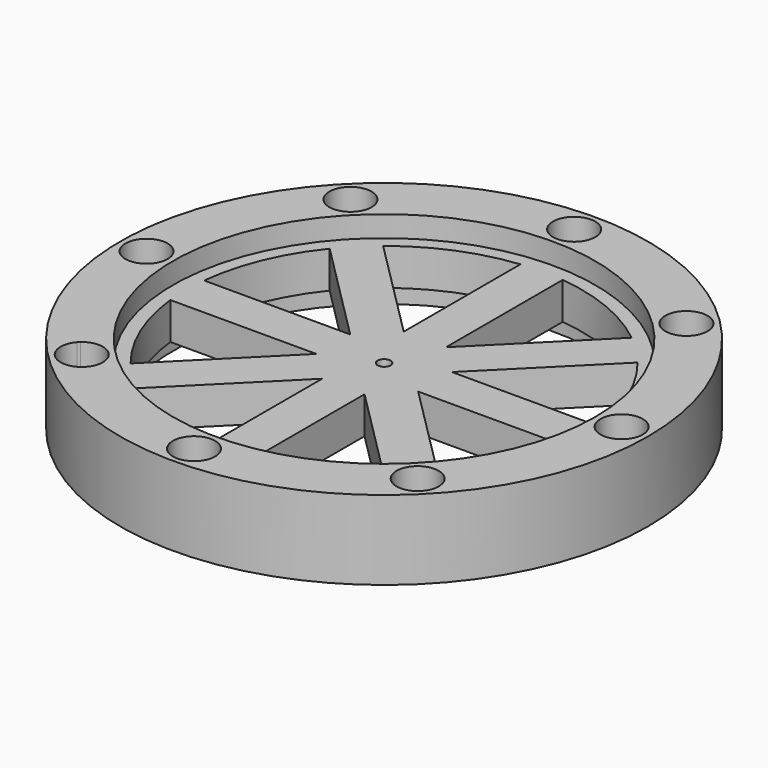
from build123d import *

# Parameters (mm, degrees)
F0_R     = 63.5
F0_R_2   = 5.08
F0_R_3   = 1.5621
F1_DEPTH = 19.05
F2_R     = 50.8
F2_R_2   = 1.5621
F3_DEPTH = 5.08
F4_R     = 50.8
F4_R_2   = 1.5621
F5_DEPTH = 5.08


with BuildPart() as f1:
    # F0 (on Top) → F1 (new body)
    with BuildSketch(Plane.XY):
        Circle(F0_R)
        with BuildLine():
            ThreePointArc((-43.7932900831, -36.6206979979), (-36.8187913893, -44.0029962675), (-44.2020942404, -37.0295610466))
            Line((-44.2020942404, -37.0295610466), (-43.7932900831, -36.6206979979))
        make_face(mode=Mode.SUBTRACT)
        with BuildLine():
            Line((-5.08, -12.2641944787), (-5.08, -47.3532915963))
            Line((-5.08, -47.3532915963), (-5.08, -50.545361805))
            ThreePointArc((-5.08, -50.545361805), (-19.4403188674, -46.9330800431), (-32.1488664849, -39.3330698488))
            Line((-32.1488664849, -39.3330698488), (-29.8917324097, -37.0759350327))
            Line((-29.8917324097, -37.0759350327), (-5.08, -12.2641944787))
        make_face(mode=Mode.SUBTRACT)
        with BuildLine():
            ThreePointArc((-39.328136569, -32.154901244), (-46.9315884756, -19.4439194393), (-50.545361805, -5.08))
            Line((-50.545361805, -5.08), (-47.3532915963, -5.08))
            Line((-47.3532915963, -5.08), (-12.2571351119, -5.08))
            Line((-12.2571351119, -5.08), (-37.0711843605, -29.8976239041))
            Line((-37.0711843605, -29.8976239041), (-39.328136569, -32.154901244))
        make_face(mode=Mode.SUBTRACT)
        with Locations((0, -57.15)):
            Circle(F0_R_2, mode=Mode.SUBTRACT)
        with BuildLine():
            ThreePointArc((44.1465586521, -36.9683134237), (36.8189179009, -44.0031227929), (43.8542666003, -36.675999857))
            Line((43.8542666003, -36.675999857), (44.1465586521, -36.9683134237))
        make_face(mode=Mode.SUBTRACT)
        with BuildLine():
            ThreePointArc((32.151702841, -39.3307513839), (19.4420111057, -46.9323790593), (5.08, -50.545361805))
            Line((5.08, -50.545361805), (5.08, -47.3532915963))
            Line((5.08, -47.3532915963), (5.08, -12.2291341303))
            Line((5.08, -12.2291341303), (29.8959656944, -37.0725216326))
            Line((29.8959656944, -37.0725216326), (32.151702841, -39.3307513839))
        make_face(mode=Mode.SUBTRACT)
        with BuildLine():
            ThreePointArc((50.545361805, -5.08), (46.9323180233, -19.4421584439), (39.3305495108, -32.1519497882))
            Line((39.3305495108, -32.1519497882), (37.0735081629, -29.8947423052))
            Line((37.0735081629, -29.8947423052), (12.2605922736, -5.08))
            Line((12.2605922736, -5.08), (47.3532915963, -5.08))
            Line((47.3532915963, -5.08), (50.545361805, -5.08))
        make_face(mode=Mode.SUBTRACT)
        with Locations((-57.15, 0)):
            Circle(F0_R_2, mode=Mode.SUBTRACT)
        with BuildLine():
            ThreePointArc((-50.545361805, 5.08), (-46.921636061, 19.4679241152), (-39.2952191809, 32.1951199645))
            Line((-39.2952191809, 32.1951199645), (-37.0394820342, 29.9368902132))
            Line((-37.0394820342, 29.9368902132), (-12.2100285331, 5.08))
            Line((-12.2100285331, 5.08), (-47.3532915963, 5.08))
            Line((-47.3532915963, 5.08), (-50.545361805, 5.08))
        make_face(mode=Mode.SUBTRACT)
        with BuildLine():
            ThreePointArc((-32.1490547855, 39.3329159407), (-19.4404312097, 46.9330335092), (-5.08, 50.545361805))
            Line((-5.08, 50.545361805), (-5.08, 47.3532915963))
            Line((-5.08, 47.3532915963), (-5.08, 12.2618686706))
            Line((-5.08, 12.2618686706), (-29.8920134376, 37.0757084577))
            Line((-29.8920134376, 37.0757084577), (-32.1490547855, 39.3329159407))
        make_face(mode=Mode.SUBTRACT)
        with Locations((-40.4111525448, 40.4111525448)):
            Circle(F0_R_2, mode=Mode.SUBTRACT)
        Circle(F0_R_3, mode=Mode.SUBTRACT)
        with BuildLine():
            ThreePointArc((39.3330592962, 32.1488793958), (46.9330768525, 19.4403265702), (50.545361805, 5.08))
            Line((50.545361805, 5.08), (47.3532915963, 5.08))
            Line((47.3532915963, 5.08), (12.2641887856, 5.08))
            Line((12.2641887856, 5.08), (37.0759252209, 29.8917445796))
            Line((37.0759252209, 29.8917445796), (39.3330592962, 32.1488793958))
        make_face(mode=Mode.SUBTRACT)
        with BuildLine():
            Line((29.8922835881, 37.0754906493), (5.08, 12.2596326602))
            Line((5.08, 12.2596326602), (5.08, 47.3532915963))
            Line((5.08, 47.3532915963), (5.08, 50.545361805))
            ThreePointArc((5.08, 50.545361805), (19.4405392034, 46.9329887764), (32.1492357966, 39.3327679892))
            Line((32.1492357966, 39.3327679892), (29.8922835881, 37.0754906493))
        make_face(mode=Mode.SUBTRACT)
        with Locations((57.15, 0)):
            Circle(F0_R_2, mode=Mode.SUBTRACT)
        with Locations((0, 57.15)):
            Circle(F0_R_2, mode=Mode.SUBTRACT)
        with Locations((40.4111525448, 40.4111525448)):
            Circle(F0_R_2, mode=Mode.SUBTRACT)
        with BuildLine():
            Line((-37.0394820342, 29.9368902132), (-39.2952191809, 32.1951199645))
            ThreePointArc((-39.2952191809, 32.1951199645), (-46.921636061, 19.4679241152), (-50.545361805, 5.08))
            Line((-50.545361805, 5.08), (-47.3532915963, 5.08))
            ThreePointArc((-47.3532915963, 5.08), (-43.9886497637, 18.2521044532), (-37.0394820342, 29.9368902132))
        make_face()
        with BuildLine():
            Line((-5.08, 47.3532915963), (-5.08, 50.545361805))
            ThreePointArc((-5.08, 50.545361805), (-19.4404312097, 46.9330335092), (-32.1490547855, 39.3329159407))
            Line((-32.1490547855, 39.3329159407), (-29.8920134376, 37.0757084577))
            ThreePointArc((-29.8920134376, 37.0757084577), (-18.2254659683, 43.9996933539), (-5.08, 47.3532915963))
        make_face()
        with BuildLine():
            Line((-47.3532915963, -5.08), (-50.545361805, -5.08))
            ThreePointArc((-50.545361805, -5.08), (-46.9315884756, -19.4439194393), (-39.328136569, -32.154901244))
            Line((-39.328136569, -32.154901244), (-37.0711843605, -29.8976239041))
            ThreePointArc((-37.0711843605, -29.8976239041), (-43.9983141632, -18.2287952371), (-47.3532915963, -5.08))
        make_face()
        with BuildLine():
            Line((-5.08, -50.545361805), (-5.08, -47.3532915963))
            ThreePointArc((-5.08, -47.3532915963), (-18.2252992134, -43.9997624264), (-29.8917324097, -37.0759350327))
            Line((-29.8917324097, -37.0759350327), (-32.1488664849, -39.3330698488))
            ThreePointArc((-32.1488664849, -39.3330698488), (-19.4403188674, -46.9330800431), (-5.08, -50.545361805))
        make_face()
        with BuildLine():
            Line((5.08, -47.3532915963), (5.08, -50.545361805))
            ThreePointArc((5.08, -50.545361805), (19.4420111057, -46.9323790593), (32.151702841, -39.3307513839))
            Line((32.151702841, -39.3307513839), (29.8959656944, -37.0725216326))
            ThreePointArc((29.8959656944, -37.0725216326), (18.2278112187, -43.9987218357), (5.08, -47.3532915963))
        make_face()
        with BuildLine():
            Line((37.0735081629, -29.8947423052), (39.3305495108, -32.1519497882))
            ThreePointArc((39.3305495108, -32.1519497882), (46.9323180233, -19.4421584439), (50.545361805, -5.08))
            Line((50.545361805, -5.08), (47.3532915963, -5.08))
            ThreePointArc((47.3532915963, -5.08), (43.9990225836, -18.2270852494), (37.0735081629, -29.8947423052))
        make_face()
        with BuildLine():
            Line((47.3532915963, 5.08), (50.545361805, 5.08))
            ThreePointArc((50.545361805, 5.08), (46.9330768525, 19.4403265702), (39.3330592962, 32.1488793958))
            Line((39.3330592962, 32.1488793958), (37.0759252209, 29.8917445796))
            ThreePointArc((37.0759252209, 29.8917445796), (43.9997594353, 18.2253064347), (47.3532915963, 5.08))
        make_face()
        with BuildLine():
            ThreePointArc((5.08, 47.3532915963), (18.2256262696, 43.9996269539), (29.8922835881, 37.0754906493))
            Line((29.8922835881, 37.0754906493), (32.1492357966, 39.3327679892))
            ThreePointArc((32.1492357966, 39.3327679892), (19.4405392034, 46.9329887764), (5.08, 50.545361805))
            Line((5.08, 50.545361805), (5.08, 47.3532915963))
        make_face()
    extrude(amount=F1_DEPTH)

    # F2 (on face) → F3 (cut)
    with BuildSketch(Plane(origin=(0, 0, 0), x_dir=(1, 0, 0), z_dir=(0, 0, -1))):
        Circle(F2_R)
        with BuildLine():
            Line((-29.8920134376, -37.0757084577), (-5.08, -12.2618686706))
            Line((-5.08, -12.2618686706), (-5.08, -47.3532915963))
            ThreePointArc((-5.08, -47.3532915963), (-18.2254659683, -43.9996933539), (-29.8920134376, -37.0757084577))
        make_face(mode=Mode.SUBTRACT)
        with BuildLine():
            Line((-47.3532915963, -5.08), (-12.2100285331, -5.08))
            Line((-12.2100285331, -5.08), (-37.0394820342, -29.9368902132))
            ThreePointArc((-37.0394820342, -29.9368902132), (-43.9886497637, -18.2521044532), (-47.3532915963, -5.08))
        make_face(mode=Mode.SUBTRACT)
        with BuildLine():
            Line((5.08, -47.3532915963), (5.08, -12.2596326602))
            Line((5.08, -12.2596326602), (29.8922835881, -37.0754906493))
            ThreePointArc((29.8922835881, -37.0754906493), (18.2256262696, -43.9996269539), (5.08, -47.3532915963))
        make_face(mode=Mode.SUBTRACT)
        with BuildLine():
            Line((37.0759252209, -29.8917445796), (12.2641887856, -5.08))
            Line((12.2641887856, -5.08), (47.3532915963, -5.08))
            ThreePointArc((47.3532915963, -5.08), (43.9997594353, -18.2253064347), (37.0759252209, -29.8917445796))
        make_face(mode=Mode.SUBTRACT)
        with BuildLine():
            Line((-37.0711843605, 29.8976239041), (-12.2571351119, 5.08))
            Line((-12.2571351119, 5.08), (-47.3532915963, 5.08))
            ThreePointArc((-47.3532915963, 5.08), (-43.9983141632, 18.2287952371), (-37.0711843605, 29.8976239041))
        make_face(mode=Mode.SUBTRACT)
        with BuildLine():
            Line((-5.08, 47.3532915963), (-5.08, 12.2641944787))
            Line((-5.08, 12.2641944787), (-29.8917324097, 37.0759350327))
            ThreePointArc((-29.8917324097, 37.0759350327), (-18.2252992134, 43.9997624264), (-5.08, 47.3532915963))
        make_face(mode=Mode.SUBTRACT)
        Circle(F2_R_2, mode=Mode.SUBTRACT)
        with BuildLine():
            ThreePointArc((37.0735081629, 29.8947423052), (43.9990225836, 18.2270852494), (47.3532915963, 5.08))
            Line((47.3532915963, 5.08), (12.2605922736, 5.08))
            Line((12.2605922736, 5.08), (37.0735081629, 29.8947423052))
        make_face(mode=Mode.SUBTRACT)
        with BuildLine():
            Line((29.8959656944, 37.0725216326), (5.08, 12.2291341303))
            Line((5.08, 12.2291341303), (5.08, 47.3532915963))
            ThreePointArc((5.08, 47.3532915963), (18.2278112187, 43.9987218357), (29.8959656944, 37.0725216326))
        make_face(mode=Mode.SUBTRACT)
        Circle(F2_R_2)
    extrude(amount=-F3_DEPTH, mode=Mode.SUBTRACT)

    # F4 (on face) → F5 (cut)
    with BuildSketch(Plane.XY.offset(19.05)):
        Circle(F4_R)
        with BuildLine():
            ThreePointArc((-5.08, -47.3532915963), (-18.2252992134, -43.9997624264), (-29.8917324097, -37.0759350327))
            Line((-29.8917324097, -37.0759350327), (-5.08, -12.2641944787))
            Line((-5.08, -12.2641944787), (-5.08, -47.3532915963))
        make_face(mode=Mode.SUBTRACT)
        with BuildLine():
            ThreePointArc((-37.0711843605, -29.8976239041), (-43.9983141632, -18.2287952371), (-47.3532915963, -5.08))
            Line((-47.3532915963, -5.08), (-12.2571351119, -5.08))
            Line((-12.2571351119, -5.08), (-37.0711843605, -29.8976239041))
        make_face(mode=Mode.SUBTRACT)
        with BuildLine():
            ThreePointArc((29.8959656944, -37.0725216326), (18.2278112187, -43.9987218357), (5.08, -47.3532915963))
            Line((5.08, -47.3532915963), (5.08, -12.2291341303))
            Line((5.08, -12.2291341303), (29.8959656944, -37.0725216326))
        make_face(mode=Mode.SUBTRACT)
        with BuildLine():
            Line((37.0735081629, -29.8947423052), (12.2605922736, -5.08))
            Line((12.2605922736, -5.08), (47.3532915963, -5.08))
            ThreePointArc((47.3532915963, -5.08), (43.9990225836, -18.2270852494), (37.0735081629, -29.8947423052))
        make_face(mode=Mode.SUBTRACT)
        with BuildLine():
            ThreePointArc((-47.3532915963, 5.08), (-43.9886497637, 18.2521044532), (-37.0394820342, 29.9368902132))
            Line((-37.0394820342, 29.9368902132), (-12.2100285331, 5.08))
            Line((-12.2100285331, 5.08), (-47.3532915963, 5.08))
        make_face(mode=Mode.SUBTRACT)
        with BuildLine():
            ThreePointArc((-29.8920134376, 37.0757084577), (-18.2254659683, 43.9996933539), (-5.08, 47.3532915963))
            Line((-5.08, 47.3532915963), (-5.08, 12.2618686706))
            Line((-5.08, 12.2618686706), (-29.8920134376, 37.0757084577))
        make_face(mode=Mode.SUBTRACT)
        Circle(F4_R_2, mode=Mode.SUBTRACT)
        with BuildLine():
            ThreePointArc((37.0759252209, 29.8917445796), (43.9997594353, 18.2253064347), (47.3532915963, 5.08))
            Line((47.3532915963, 5.08), (12.2641887856, 5.08))
            Line((12.2641887856, 5.08), (37.0759252209, 29.8917445796))
        make_face(mode=Mode.SUBTRACT)
        with BuildLine():
            ThreePointArc((5.08, 47.3532915963), (18.2256262696, 43.9996269539), (29.8922835881, 37.0754906493))
            Line((29.8922835881, 37.0754906493), (5.08, 12.2596326602))
            Line((5.08, 12.2596326602), (5.08, 47.3532915963))
        make_face(mode=Mode.SUBTRACT)
    extrude(amount=-F5_DEPTH, mode=Mode.SUBTRACT)


solid = f1.part
